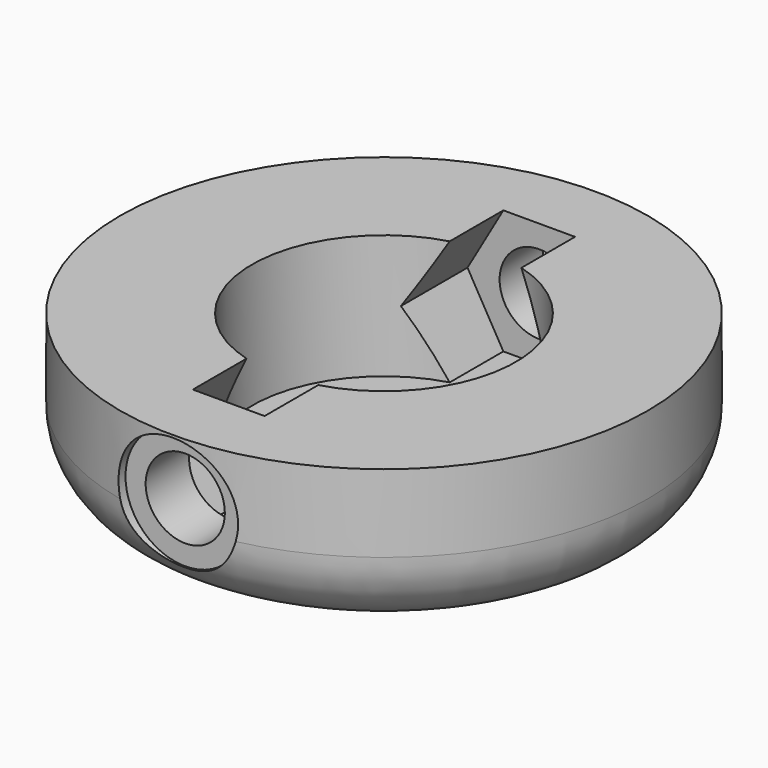
from build123d import *

# Parameters (mm, degrees)
F0_R      = 17
F1_DEPTH  = 10
F2_R      = 8.5
F3_DEPTH  = 8
F4_R      = 6.5
F5_DEPTH  = 2.001
F7_DEPTH  = 12.5
F10_R     = 3.85
F11_DEPTH = 1.5
F12_R     = 3.85
F13_DEPTH = 1.5
F15_R     = 2.55
F16_DEPTH = 34.5010001


# Not quite as in the source:
# - a fillet or chamfer that OpenCascade refuses, or shapes differently, is made with other operations: its cross-section is extruded or revolved along the edge and cut away or added


with BuildPart() as f1:
    # F0 (on Top) → F1 (new body)
    with BuildSketch(Plane.XY):
        Circle(F0_R)
    extrude(amount=F1_DEPTH)

    # F2 (on face) → F3 (cut)
    with BuildSketch(Plane.XY.offset(10)):
        Circle(F2_R)
    extrude(amount=-F3_DEPTH, mode=Mode.SUBTRACT)

    # F4 (on face) → F5 (cut, through all)
    with BuildSketch(Plane.XY.offset(2)):
        Circle(F4_R)
    extrude(amount=-F5_DEPTH, mode=Mode.SUBTRACT)

    # F6 (on Front) → F7 (cut, symmetric)
    with BuildSketch(Plane.XZ):
        Polygon((4.6188021535, 6), (2.3094010768, 10), (-2.3094010768, 10), (-4.6188021535, 6), (-2.3094010768, 2), (2.3094010768, 2), align=None)
    extrude(amount=F7_DEPTH, both=True, mode=Mode.SUBTRACT)

    # F10 (on offset) → F11 (cut)
    with BuildSketch(Plane.XZ.offset(17.5)):
        with Locations((0, 6)):
            Circle(F10_R)
    extrude(amount=-F11_DEPTH, mode=Mode.SUBTRACT)

    # F12 (on offset) → F13 (cut)
    with BuildSketch(Plane.XZ.offset(-17.5)):
        with Locations((0, 6)):
            Circle(F12_R)
    extrude(amount=F13_DEPTH, mode=Mode.SUBTRACT)

    # F14: fillet of radius 5 on 1 edges, made by hand

    # F14_s1 → F14_t2 (revolve, cut)
    with BuildSketch(Plane.XZ):
        with BuildLine():
            ThreePointArc((17, 5), (15.5355339059, 1.4644660941), (12, 0))
            Line((12, 0), (17, 0))
            Line((17, 0), (17, 5))
        make_face()
    revolve(axis=Axis((0, 0, 0), (0, 0, 1)), mode=Mode.SUBTRACT)

    # F15 (on offset) → F16 (cut, through all)
    with BuildSketch(Plane.XZ.offset(17.5)):
        with Locations((0, 6)):
            Circle(F15_R)
    extrude(amount=-F16_DEPTH, mode=Mode.SUBTRACT)


solid = f1.part
